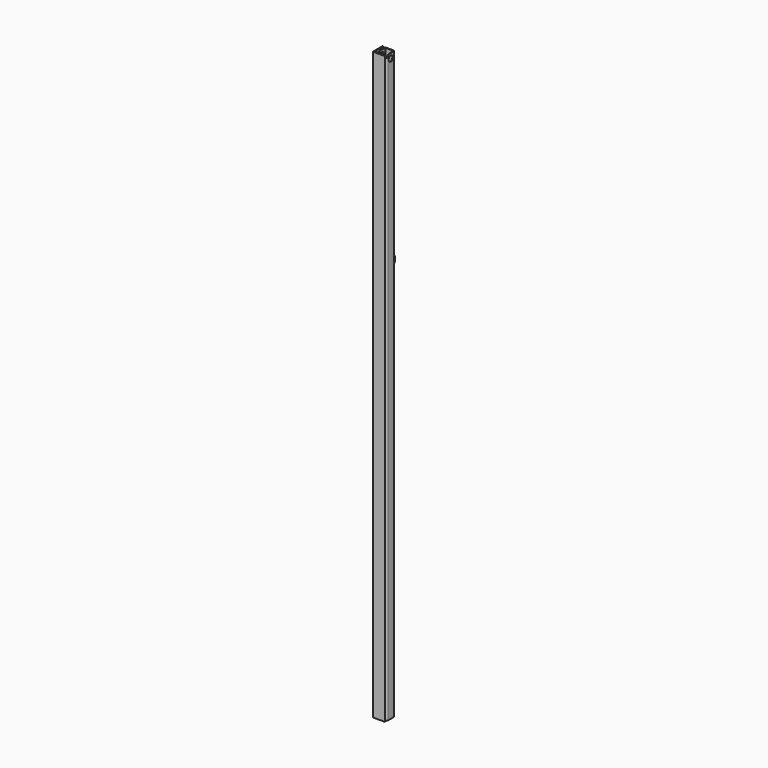
from build123d import *

# Parameters (mm, degrees)
F1_DEPTH      = 6096
F1_DEPTH_BACK = 50.8
F2_DEPTH      = 50.8
F2_DEPTH_BACK = 6096
F3_R          = 15.875
F4_DEPTH      = 9.526
F3_R_2        = 28.575
F3_R_3        = 19.05
F5_DEPTH      = 120.651
F5_DEPTH_BACK = 9.526
F7_R          = 19.05
F8_DEPTH      = 12.7
F9_R          = 6.35
F11_DEPTH     = 130.176


# Not quite as in the source:
# - the program builds the solid bodies; features that only make, move or delete a surface that nothing else refers to are left out


with BuildPart() as f1:
    # F12 (on Top) → F1 (new body, two sides)
    with BuildSketch(Plane.XY) as f1_sk:
        with BuildLine():
            ThreePointArc((50.8, 38.1), (47.0802561211, 47.0802561211), (38.1, 50.8))
            Line((38.1, 50.8), (-38.1, 50.8))
            ThreePointArc((-38.1, 50.8), (-47.0802561211, 47.0802561211), (-50.8, 38.1))
            Line((-50.8, 38.1), (-50.8, -38.1))
            ThreePointArc((-50.8, -38.1), (-47.0802561211, -47.0802561211), (-38.1, -50.8))
            Line((-38.1, -50.8), (38.1, -50.8))
            ThreePointArc((38.1, -50.8), (47.0802561211, -47.0802561211), (50.8, -38.1))
            Line((50.8, -38.1), (50.8, 38.1))
        make_face()
        with BuildLine():
            ThreePointArc((-44.45, 38.1), (-42.5901280605, 42.5901280605), (-38.1, 44.45))
            Line((-38.1, 44.45), (38.1, 44.45))
            ThreePointArc((38.1, 44.45), (42.5901280605, 42.5901280605), (44.45, 38.1))
            Line((44.45, 38.1), (44.45, -38.1))
            ThreePointArc((44.45, -38.1), (42.5901280605, -42.5901280605), (38.1, -44.45))
            Line((38.1, -44.45), (-38.1, -44.45))
            ThreePointArc((-38.1, -44.45), (-42.5901280605, -42.5901280605), (-44.45, -38.1))
            Line((-44.45, -38.1), (-44.45, 38.1))
        make_face(mode=Mode.SUBTRACT)
    extrude(amount=-F1_DEPTH)
    extrude(f1_sk.sketch, amount=F1_DEPTH_BACK)


with BuildPart() as f2:
    # F12 (on Top) → F2 (new body, two sides)
    with BuildSketch(Plane.XY) as f2_sk:
        with BuildLine():
            Line((-69.85, -53.975), (-69.85, 44.45))
            ThreePointArc((-69.85, 44.45), (-72.6398079092, 51.1851920908), (-79.375, 53.975))
            Line((-79.375, 53.975), (-79.375, -73.025))
            Line((-79.375, -73.025), (47.625, -73.025))
            ThreePointArc((47.625, -73.025), (44.8351920908, -66.2898079092), (38.1, -63.5))
            Line((38.1, -63.5), (-60.325, -63.5))
            ThreePointArc((-60.325, -63.5), (-67.0601920908, -60.7101920908), (-69.85, -53.975))
        make_face()
    extrude(amount=F2_DEPTH)
    extrude(f2_sk.sketch, amount=-F2_DEPTH_BACK)

    # F3 (on face) → F4 (cut, through all)
    with BuildSketch(Plane.YZ.offset(-69.85)):
        with Locations((0, -4792.820472761)):
            Circle(F3_R)
    extrude(amount=-F4_DEPTH, mode=Mode.SUBTRACT)


with BuildPart() as f5_tool:
    # F3 (on face) → F5 (new body, two sides)
    with BuildSketch(Plane.YZ.offset(-69.85)) as f5_sk:
        Circle(F3_R_2)
        Circle(F3_R_3, mode=Mode.SUBTRACT)
        Circle(F3_R_3)
    extrude(amount=F5_DEPTH)
    extrude(f5_sk.sketch, amount=-F5_DEPTH_BACK)


with BuildPart() as f1_1:
    add(f1.part)

    # F5: cut by f5_tool
    add(f5_tool.part, mode=Mode.SUBTRACT)

    # F10 (on face) → F11 (cut, through all)
    with BuildSketch(Plane.YZ.offset(50.8)):
        with BuildLine():
            Line((-38.1, 50.8), (-38.1, 33.6010416505))
            ThreePointArc((-38.1, 33.6010416505), (-20.9010416505, 46.3010416505), (0, 50.8))
            Line((0, 50.8), (-38.1, 50.8))
        make_face()
        with BuildLine():
            Line((-50.8, 24.5934442484), (-44.45, 24.5934442484))
            ThreePointArc((-44.45, 24.5934442484), (-41.5199931086, 29.2699534038), (-38.1, 33.6010416505))
            Line((-38.1, 33.6010416505), (-38.1, 50.8))
            Line((-38.1, 50.8), (-50.8, 50.8))
            Line((-50.8, 50.8), (-50.8, 24.5934442484))
        make_face()
    extrude(amount=-F11_DEPTH, mode=Mode.SUBTRACT)


with BuildPart() as f2_1:
    add(f2.part)

    # F5: cut by f5_tool
    add(f5_tool.part, mode=Mode.SUBTRACT)


with BuildPart() as f8:
    # F7 (on face) → F8 (new body)
    with BuildSketch(Plane(origin=(-50.8, 0, 0), x_dir=(0, -1, 0), z_dir=(-1, 0, 0))):
        with BuildLine():
            Line((-38.1, -2165.878324814), (-38.1, -1880.2239560519))
            Line((-38.1, -1880.2239560519), (-107.95, -1880.2239560519))
            ThreePointArc((-107.95, -1880.2239560519), (-176.6212263011, -1923.3981679718), (-167.4754951972, -2003.9965891672))
            Line((-167.4754951972, -2003.9965891672), (-38.1, -2165.878324814))
        make_face()
        with Locations((-107.95, -1956.4239560519)):
            Circle(F7_R, mode=Mode.SUBTRACT)
        Polygon((38.1, -2261.2239560519), (38.1, -1880.2239560519), (-38.1, -1880.2239560519), (-38.1, -2165.878324814), align=None)
    extrude(amount=F8_DEPTH)

    # F9
    f9_edges = [f8.edges().sort_by_distance(p)[0] for p in [
        (-57.15, -38.1, -1880.223956),
        (-57.15, -38.1, -2261.223956),
    ]]
    fillet(f9_edges, radius=F9_R)


solid = Compound([f1_1.part, f2_1.part, f8.part])
